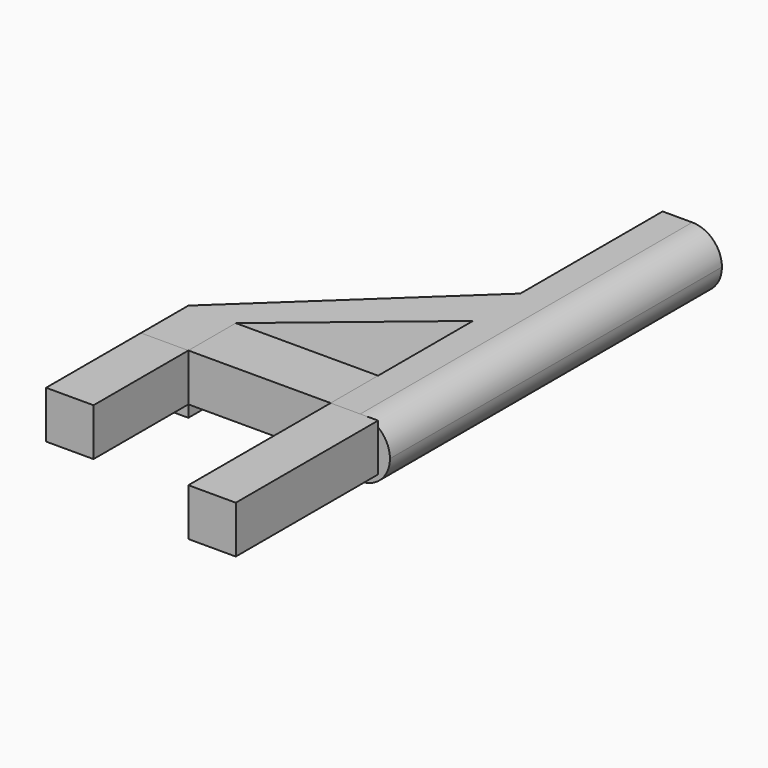
from build123d import *

# Parameters (mm, degrees)
F0_W     = 4
F0_H     = 4
F1_DEPTH = 10
F2_DEPTH = 15
F0_W_2   = 12
F3_DEPTH = 5
F4_W     = 4
F4_H     = 5
F4_W_2   = 5
F5_DEPTH = 5
F6_R     = 2.49999


# Not quite as in the source:
# - a fillet or chamfer is up to 0.001 mm smaller than in the source, because OpenCascade refuses the exact size


with BuildPart() as f1:
    # F0 (on Front) → F1 (new body)
    with BuildSketch(Plane.XZ):
        with Locations((2, 2)):
            Rectangle(F0_W, F0_H)
    extrude(amount=F1_DEPTH)


with BuildPart() as f2:
    # F0 (on Front) → F2 (new body)
    with BuildSketch(Plane.XZ):
        with Locations((18, 2)):
            Rectangle(F0_W, F0_H)
    extrude(amount=F2_DEPTH)


with BuildPart() as f3:
    # F0 (on Front) → F3 (new body)
    with BuildSketch(Plane.XZ):
        with Locations((10, 2)):
            Rectangle(F0_W_2, F0_H)
    extrude(amount=-F3_DEPTH)


with BuildPart() as f5:
    # F4 (on face) → F5 (new body)
    with BuildSketch(Plane.XY.offset(4)):
        Polygon((16, 15), (16, 5), (21, 5), (21, 35), (16, 35), (16, 20), align=None)
        with Locations((2, 2.5)):
            Rectangle(F4_W, F4_H)
        Polygon((4, 5), (16, 15), (16, 20), (0, 5), align=None)
        with Locations((18.5, 2.5)):
            Rectangle(F4_W_2, F4_H)
    extrude(amount=-F5_DEPTH)

    # F6 (radius 2.5 in the source; OpenCascade refuses exactly that, so slightly less here)
    f6_edges = [f5.edges().sort_by_distance(p)[0] for p in [
        (21, 17.5, -1),
        (21, 17.5, 4),
    ]]
    fillet(f6_edges, radius=F6_R)


solid = Compound([f1.part, f2.part, f3.part, f5.part])
